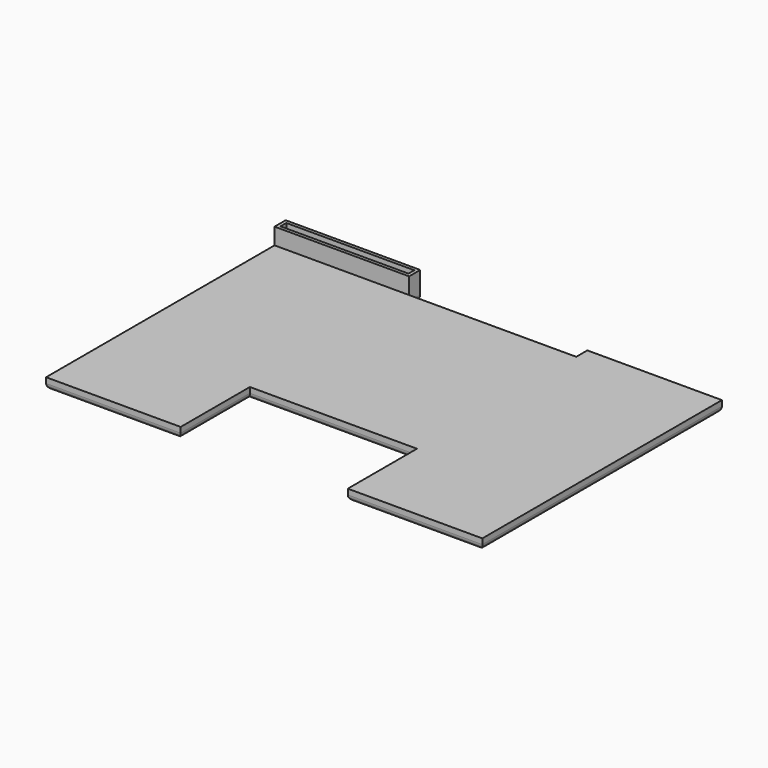
from build123d import *

# Parameters (mm, degrees)
F1_DEPTH     = 2
F2_W         = 23.3004903048
F2_H         = 1.3265815725
F3_DEPTH     = 2
F2_W_2       = 24.5004919916
F2_H_2       = 2.5265832593
F4_DEPTH     = 3
F5_T1_DEPTH  = 29.5004919916
F5_T3_DEPTH  = 59.5122700134
F5_T5_DEPTH  = 5.0265832593
F5_T7_DEPTH  = 30.4185097339
F5_T9_DEPTH  = 18.246874844
F5_T11_DEPTH = 29.5004919916
F5_T17_DEPTH = 7.5265832593
F5_T21_DEPTH = 32.9185097339
F5_T28_DEPTH = 32.9185097339
F5_T32_DEPTH = 7.5265832593
F5_T39_DEPTH = 20.746874844
F5_T43_DEPTH = 32.9185097339
F5_T50_DEPTH = 32.9185097339
F5_T54_DEPTH = 20.746874844


# Not quite as in the source:
# - a fillet or chamfer that OpenCascade refuses, or shapes differently, is made with other operations: its cross-section is extruded or revolved along the edge and cut away or added


with BuildPart() as f1:
    # F0 (on Top) → F1 (new body)
    with BuildSketch(Plane.XY):
        Polygon((25.1509650471, -26.6069659193), (25.1509650471, 27.9053040941), (0.6504730554, 27.9053040941), (0.6504730554, 25.3787208349), (-29.7680366784, 25.3787208349), (-29.7680366784, 27.9053040941), (-54.2685286701, 27.9053040941), (-54.2685286701, -26.6069659193), (-29.7680366784, -26.6069659193), (-29.7680366784, -10.8600910753), (0.6504730554, -10.8600910753), (0.6504730554, -26.6069659193), align=None)
    extrude(amount=F1_DEPTH)

    # F0 (on Top) + F2 (on face) → F3 (cut)
    with BuildSketch(Plane.XY):
        Polygon((25.1509650471, -26.6069659193), (25.1509650471, 27.9053040941), (0.6504730554, 27.9053040941), (0.6504730554, 25.3787208349), (-29.7680366784, 25.3787208349), (-29.7680366784, 27.9053040941), (-54.2685286701, 27.9053040941), (-54.2685286701, -26.6069659193), (-29.7680366784, -26.6069659193), (-29.7680366784, -10.8600910753), (0.6504730554, -10.8600910753), (0.6504730554, -26.6069659193), align=None)
    with BuildSketch(Plane.XY.offset(2)):
        with Locations((-42.0182826743, 26.6420124645)):
            Rectangle(F2_W, F2_H)
    extrude(amount=-F3_DEPTH, mode=Mode.SUBTRACT)

    # F2 (on face) → F4 (join)
    with BuildSketch(Plane.XY.offset(2)):
        with Locations((-42.0182826743, 26.6420124645)):
            Rectangle(F2_W_2, F2_H_2)
        with Locations((-42.0182826743, 26.6420124645)):
            Rectangle(F2_W, F2_H, mode=Mode.SUBTRACT)
    extrude(amount=F4_DEPTH)

    # F5: fillet of radius 1 on 12 edges, made by hand

    # F5_s2 → F5_t1 (cut)
    with BuildSketch(Plane.YZ.offset(-56.7685286701)):
        with BuildLine():
            ThreePointArc((-25.6069659193, 0), (-26.3140727005, 0.2928932188), (-26.6069659193, 1))
            Line((-26.6069659193, 1), (-26.6069659193, 0))
            Line((-26.6069659193, 0), (-25.6069659193, 0))
        make_face()
        with BuildLine():
            ThreePointArc((26.9053040941, 0), (27.6124108753, 0.2928932188), (27.9053040941, 1))
            Line((27.9053040941, 1), (27.9053040941, 0))
            Line((27.9053040941, 0), (26.9053040941, 0))
        make_face()
    extrude(amount=F5_T1_DEPTH, mode=Mode.SUBTRACT)

    # F5_s4 → F5_t3 (cut)
    with BuildSketch(Plane.XZ.offset(-30.4053040941)):
        with BuildLine():
            ThreePointArc((-54.2685286701, 1), (-53.9756354513, 0.2928932188), (-53.2685286701, 0))
            Line((-53.2685286701, 0), (-54.2685286701, 0))
            Line((-54.2685286701, 0), (-54.2685286701, 1))
        make_face()
        with BuildLine():
            ThreePointArc((24.1509650471, 0), (24.8580718283, 0.2928932188), (25.1509650471, 1))
            Line((25.1509650471, 1), (25.1509650471, 0))
            Line((25.1509650471, 0), (24.1509650471, 0))
        make_face()
    extrude(amount=F5_T3_DEPTH, mode=Mode.SUBTRACT)

    # F5_s6 → F5_t5 (cut)
    with BuildSketch(Plane.XZ.offset(-30.4053040941)):
        with BuildLine():
            ThreePointArc((-30.7680366784, 0), (-30.0609298972, 0.2928932188), (-29.7680366784, 1))
            Line((-29.7680366784, 1), (-29.7680366784, 0))
            Line((-29.7680366784, 0), (-30.7680366784, 0))
        make_face()
        with BuildLine():
            ThreePointArc((1.6504730554, 0), (0.9433662742, 0.2928932188), (0.6504730554, 1))
            Line((0.6504730554, 1), (0.6504730554, 0))
            Line((0.6504730554, 0), (1.6504730554, 0))
        make_face()
    extrude(amount=F5_T5_DEPTH, mode=Mode.SUBTRACT)

    # F5_s8 → F5_t7 (cut)
    with BuildSketch(Plane.YZ.offset(-29.7680366784)):
        with BuildLine():
            ThreePointArc((24.3787208349, 0), (25.085827616, 0.2928932188), (25.3787208349, 1))
            Line((25.3787208349, 1), (25.3787208349, 0))
            Line((25.3787208349, 0), (24.3787208349, 0))
        make_face()
        with BuildLine():
            ThreePointArc((-9.8600910753, 0), (-10.5671978565, 0.2928932188), (-10.8600910753, 1))
            Line((-10.8600910753, 1), (-10.8600910753, 0))
            Line((-10.8600910753, 0), (-9.8600910753, 0))
        make_face()
    extrude(amount=F5_T7_DEPTH, mode=Mode.SUBTRACT)

    # F5_s10 → F5_t9 (cut)
    with BuildSketch(Plane.XZ.offset(10.8600910753)):
        with BuildLine():
            ThreePointArc((-30.7680366784, 0), (-30.0609298972, 0.2928932188), (-29.7680366784, 1))
            Line((-29.7680366784, 1), (-29.7680366784, 0))
            Line((-29.7680366784, 0), (-30.7680366784, 0))
        make_face()
        with BuildLine():
            ThreePointArc((1.6504730554, 0), (0.9433662742, 0.2928932188), (0.6504730554, 1))
            Line((0.6504730554, 1), (0.6504730554, 0))
            Line((0.6504730554, 0), (1.6504730554, 0))
        make_face()
    extrude(amount=F5_T9_DEPTH, mode=Mode.SUBTRACT)

    # F5_s12 → F5_t11 (cut)
    with BuildSketch(Plane.YZ.offset(-1.8495269446)):
        with BuildLine():
            ThreePointArc((-25.6069659193, 0), (-26.3140727005, 0.2928932188), (-26.6069659193, 1))
            Line((-26.6069659193, 1), (-26.6069659193, 0))
            Line((-26.6069659193, 0), (-25.6069659193, 0))
        make_face()
        with BuildLine():
            ThreePointArc((26.9053040941, 0), (27.6124108753, 0.2928932188), (27.9053040941, 1))
            Line((27.9053040941, 1), (27.9053040941, 0))
            Line((27.9053040941, 0), (26.9053040941, 0))
        make_face()
    extrude(amount=F5_T11_DEPTH, mode=Mode.SUBTRACT)


with BuildPart() as f5_tool15:
    # F5_s16 → F5_t17 (new body)
    with BuildSketch(Plane.XZ.offset(-22.8787208349)):
        with BuildLine():
            ThreePointArc((-30.7680366784, 0), (-30.0609298972, 0.2928932188), (-29.7680366784, 1))
            Line((-29.7680366784, 1), (-29.7680366784, 0))
            Line((-29.7680366784, 0), (-30.7680366784, 0))
        make_face()
    extrude(amount=-F5_T17_DEPTH)

    split(bisect_by=Plane.XZ.offset(-25.3787208349), keep=Keep.TOP)


with BuildPart() as f5_tool19:
    # F5_s20 → F5_t21 (new body)
    with BuildSketch(Plane.YZ.offset(0.6504730554)):
        with BuildLine():
            ThreePointArc((24.3787208349, 0), (25.085827616, 0.2928932188), (25.3787208349, 1))
            Line((25.3787208349, 1), (25.3787208349, 0))
            Line((25.3787208349, 0), (24.3787208349, 0))
        make_face()
    extrude(amount=-F5_T21_DEPTH)

    split(bisect_by=Plane.YZ.offset(-29.7680366784), keep=Keep.BOTTOM)


with BuildPart() as f5_tool15_1:
    add(f5_tool15.part)

    # F5_t23: intersect F5_tool19
    add(f5_tool19.part, mode=Mode.INTERSECT)


with BuildPart() as f1_1:
    add(f1.part)

    # F5_t13: cut F5_tool15
    add(f5_tool15_1.part, mode=Mode.SUBTRACT)


with BuildPart() as f5_tool26:
    # F5_s27 → F5_t28 (new body)
    with BuildSketch(Plane.YZ.offset(3.1504730554)):
        with BuildLine():
            ThreePointArc((24.3787208349, 0), (25.085827616, 0.2928932188), (25.3787208349, 1))
            Line((25.3787208349, 1), (25.3787208349, 0))
            Line((25.3787208349, 0), (24.3787208349, 0))
        make_face()
    extrude(amount=-F5_T28_DEPTH)

    split(bisect_by=Plane.YZ.offset(0.6504730554), keep=Keep.TOP)


with BuildPart() as f5_tool30:
    # F5_s31 → F5_t32 (new body)
    with BuildSketch(Plane.XZ.offset(-30.4053040941)):
        with BuildLine():
            ThreePointArc((1.6504730554, 0), (0.9433662742, 0.2928932188), (0.6504730554, 1))
            Line((0.6504730554, 1), (0.6504730554, 0))
            Line((0.6504730554, 0), (1.6504730554, 0))
        make_face()
    extrude(amount=F5_T32_DEPTH)

    split(bisect_by=Plane.XZ.offset(-25.3787208349), keep=Keep.TOP)


with BuildPart() as f5_tool26_1:
    add(f5_tool26.part)

    # F5_t34: intersect F5_tool30
    add(f5_tool30.part, mode=Mode.INTERSECT)


with BuildPart() as f1_2:
    add(f1_1.part)

    # F5_t24: cut F5_tool26
    add(f5_tool26_1.part, mode=Mode.SUBTRACT)


with BuildPart() as f5_tool37:
    # F5_s38 → F5_t39 (new body)
    with BuildSketch(Plane.XZ.offset(29.1069659193)):
        with BuildLine():
            ThreePointArc((-30.7680366784, 0), (-30.0609298972, 0.2928932188), (-29.7680366784, 1))
            Line((-29.7680366784, 1), (-29.7680366784, 0))
            Line((-29.7680366784, 0), (-30.7680366784, 0))
        make_face()
    extrude(amount=-F5_T39_DEPTH)

    split(bisect_by=Plane.XZ.offset(10.8600910753), keep=Keep.BOTTOM)


with BuildPart() as f5_tool41:
    # F5_s42 → F5_t43 (new body)
    with BuildSketch(Plane.YZ.offset(-32.2680366784)):
        with BuildLine():
            ThreePointArc((-9.8600910753, 0), (-10.5671978565, 0.2928932188), (-10.8600910753, 1))
            Line((-10.8600910753, 1), (-10.8600910753, 0))
            Line((-10.8600910753, 0), (-9.8600910753, 0))
        make_face()
    extrude(amount=F5_T43_DEPTH)

    split(bisect_by=Plane.YZ.offset(-29.7680366784), keep=Keep.BOTTOM)


with BuildPart() as f5_tool37_1:
    add(f5_tool37.part)

    # F5_t45: intersect F5_tool41
    add(f5_tool41.part, mode=Mode.INTERSECT)


with BuildPart() as f1_3:
    add(f1_2.part)

    # F5_t35: cut F5_tool37
    add(f5_tool37_1.part, mode=Mode.SUBTRACT)


with BuildPart() as f5_tool48:
    # F5_s49 → F5_t50 (new body)
    with BuildSketch(Plane.YZ.offset(-29.7680366784)):
        with BuildLine():
            ThreePointArc((-9.8600910753, 0), (-10.5671978565, 0.2928932188), (-10.8600910753, 1))
            Line((-10.8600910753, 1), (-10.8600910753, 0))
            Line((-10.8600910753, 0), (-9.8600910753, 0))
        make_face()
    extrude(amount=F5_T50_DEPTH)

    split(bisect_by=Plane.YZ.offset(0.6504730554), keep=Keep.TOP)


with BuildPart() as f5_tool52:
    # F5_s53 → F5_t54 (new body)
    with BuildSketch(Plane.XZ.offset(8.3600910753)):
        with BuildLine():
            ThreePointArc((1.6504730554, 0), (0.9433662742, 0.2928932188), (0.6504730554, 1))
            Line((0.6504730554, 1), (0.6504730554, 0))
            Line((0.6504730554, 0), (1.6504730554, 0))
        make_face()
    extrude(amount=F5_T54_DEPTH)

    split(bisect_by=Plane.XZ.offset(10.8600910753), keep=Keep.BOTTOM)


with BuildPart() as f5_tool48_1:
    add(f5_tool48.part)

    # F5_t56: intersect F5_tool52
    add(f5_tool52.part, mode=Mode.INTERSECT)


with BuildPart() as f1_4:
    add(f1_3.part)

    # F5_t46: cut F5_tool48
    add(f5_tool48_1.part, mode=Mode.SUBTRACT)


solid = f1_4.part
